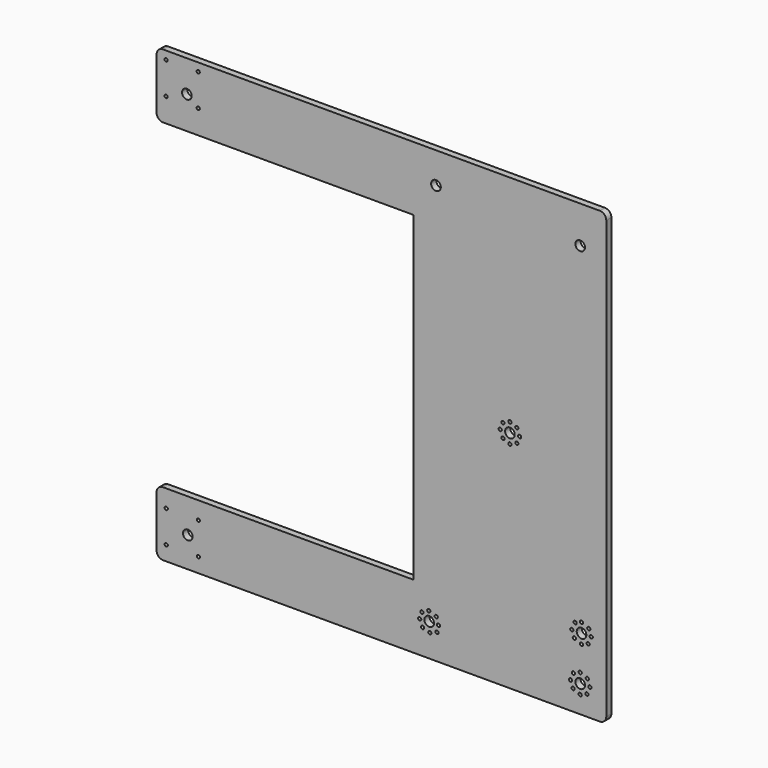
from build123d import *

# Parameters (mm, degrees)
F1_DEPTH = 5.08
F3_D     = 7.62
F4_R     = 5.08
F6_D     = 2.54
F8_D     = 7.62
F10_D    = 2.54
F12_D    = 2.54
F14_D    = 7.62
F16_D    = 7.62


# Not quite as in the source:
# - a feature names something its author has since deleted; it is built from what else it names


with BuildPart() as f1:
    # F0 (on Front) → F1 (new body)
    with BuildSketch(Plane.XZ):
        Polygon((27.4981856346, 177.8), (-177.8, 177.8), (-177.8, 127), (25.4, 127), (25.4, -127), (-177.8, -127), (-177.8, -177.8), (25.4, -177.8), (177.8, -177.8), (177.8, 177.8), align=None)
    extrude(amount=F1_DEPTH)

    # F3 (through all)
    with Locations(Plane.XZ.offset(5.08)):
        with Locations((-153.8637131453, 152.8165191412), (101.6, 0), (-153.1574577093, -153.8859605789), (157.1783274412, -156.3732177019), (157.1783274412, 148.4267822981)):
            Hole(F3_D / 2)

    # F4
    f4_edges = [f1.edges().sort_by_distance(p)[0] for p in [
        (177.8, -2.54, 177.8),
        (-177.8, -2.54, 177.8),
        (-177.8, -2.54, 127),
        (-177.8, -2.54, -127),
        (-177.8, -2.54, -177.8),
        (177.8, -2.54, -177.8),
    ]]
    fillet(f4_edges, radius=F4_R)

    # F6 (through all)
    with Locations(Plane.XZ.offset(5.08)):
        with Locations((93.9038, 0), (101.6, 7.6962), (109.2962, 0), (101.6, -7.6962), (-170.1568275641, -140.8739216598), (-144.7568275641, -140.8739216598), (-170.1568275641, -166.2739216598), (-144.7568275641, -166.2739216598), (157.1783274412, -148.6770177019), (151.850887514, -150.8189510301), (162.4951099118, -161.9376870028), (157.1783274412, -164.0694177019), (-170.2933631182, 171.3147368595), (-144.8933631182, 171.3147368595), (-144.8933631182, 145.9147368595), (-170.2933631182, 145.9147368595), (96.0876377272, 5.3707873365), (107.050479993, 5.433577301), (107.1167234014, -5.3663076089), (96.1674041077, -5.4514581821), (149.4821274412, -156.3732177019), (151.5333356816, -161.6044281234), (164.8745274412, -156.3732177019), (162.7891082701, -151.1053307507)):
            Hole(F6_D / 2)

    # F8 (through all)
    with Locations(Plane(origin=(0, 0, 0), x_dir=(-1, 0, 0), z_dir=(0, 1, 0))):
        with Locations((-158.2407057285, -121.0239678621)):
            Hole(F8_D / 2)

    # F10 (through all)
    with Locations(Plane.XZ.offset(5.08)):
        with Locations((165.9369057285, -121.0239678621), (164.0052020571, -115.9247447333), (163.4948166475, -126.6476510761), (158.2407057285, -128.7201678621), (152.5501607373, -126.2055884718), (150.5445057285, -121.0239678621), (153.1963041185, -115.2114377042), (158.2407057285, -113.3277678621)):
            Hole(F10_D / 2)

    # F12 (through all)
    with Locations(Plane.XZ.offset(5.08)):
        with Locations((32.0593006909, -147.3129242659), (37.4611556555, -144.6748753268), (43.3156022713, -146.8128675346), (45.0811556555, -152.2948753268), (43.8902415335, -157.5409770012), (38.2883101702, -159.6900522709), (32.5446762145, -157.8294336796), (30.2795823663, -152.5711715221)):
            Hole(F12_D / 2)

    # F14 (through all)
    with Locations(Plane.XZ.offset(5.08)):
        with Locations((37.7828851342, -151.951700449)):
            Hole(F14_D / 2)

    # F16 (through all)
    with Locations(Plane.XZ.offset(5.08)):
        with Locations((43.1287847459, 153.2645523548)):
            Hole(F16_D / 2)


solid = f1.part
